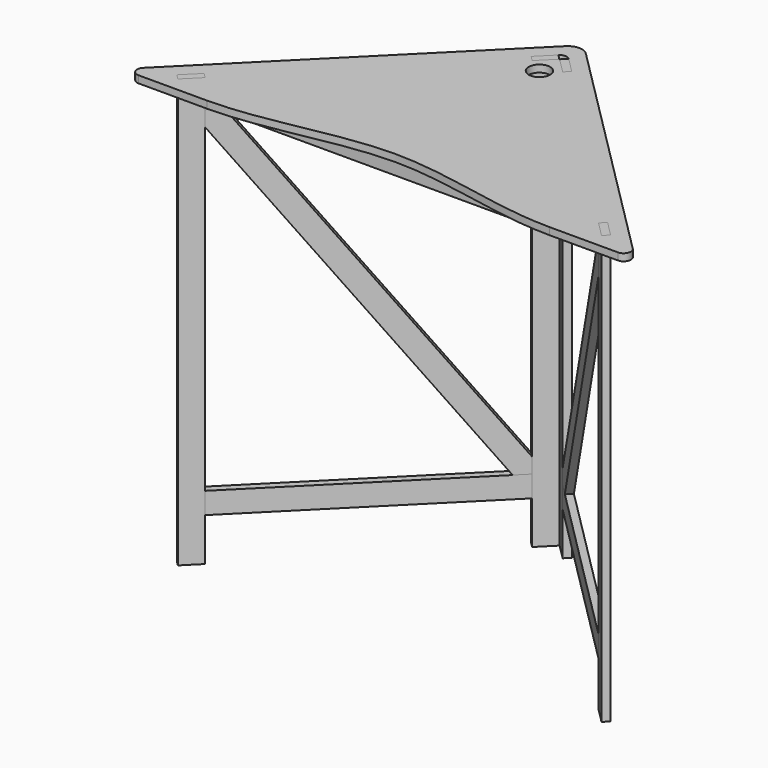
from build123d import *

# Parameters (mm, degrees)
F3_DEPTH  = 12.7
F2_R      = 19.05
F4_DEPTH  = 12.7
F5_DEPTH  = 762
F6_W      = 12.7
F6_H      = 38.1
F7_DEPTH  = 457.1994660567
F9_DEPTH  = 12.7
F11_W     = 12.7
F11_H     = 38.1
F12_REACH = 479.401414142
F13_REACH = 479.401414142


with BuildPart() as f3:
    # F1 (on Top) → F3 (new body)
    with BuildSketch(Plane.XY):
        with BuildLine():
            Line((435.5197438789, 21.6802561211), (17.9605122421, 439.2394877579))
            ThreePointArc((17.9605122421, 439.2394877579), (0, 446.6789755157), (-17.9605122421, 439.2394877579))
            Line((-17.9605122421, 439.2394877579), (-435.5197438789, 21.6802561211))
            ThreePointArc((-435.5197438789, 21.6802561211), (-438.2727578208, 7.839920409), (-426.5394877579, 0))
            Line((-426.5394877579, 0), (-304.8, 0))
            add(Edge.make_bspline(
                [(-304.8, 0), (-203.2, 0), (0, 76.2), (203.2, 0), (304.8, 0)],
                knots=[0, 0, 0, 0, 0.5, 1, 1, 1, 1], degree=3))
            Line((304.8, 0), (426.5394877579, 0))
            ThreePointArc((426.5394877579, 0), (438.2727578208, 7.839920409), (435.5197438789, 21.6802561211))
        make_face()
    extrude(amount=-F3_DEPTH)

    # F2 (on Top) → F4 (cut, through all)
    with BuildSketch(Plane.XY):
        Polygon((-27.1947683632, 376.1236949104), (-0.254, 403.0644632736), (-9.2342561211, 412.0447193947), (-36.1750244843, 385.1039510314), align=None)
        with BuildLine():
            Line((-9.2342561211, 412.0447193947), (-0.254, 403.0644632736))
            ThreePointArc((-0.254, 403.0644632736), (0, 403.1696735184), (0.254, 403.0644632736))
            Line((0.254, 403.0644632736), (9.2342561211, 412.0447193947))
            ThreePointArc((9.2342561211, 412.0447193947), (0, 415.8696735184), (-9.2342561211, 412.0447193947))
        make_face()
        Polygon((9.2342561211, 412.0447193947), (0.254, 403.0644632736), (27.1947683632, 376.1236949104), (36.1750244843, 385.1039510314), align=None)
        Polygon((-358.9697835442, 61.3210244843), (-385.9105519074, 34.3802561211), (-376.9302957863, 25.4), (-349.9895274231, 52.3407683632), align=None)
        Polygon((358.9697835442, 61.3210244843), (349.9895274231, 52.3407683632), (376.9302957863, 25.4), (385.9105519074, 34.3802561211), align=None)
        with Locations((0, 358.4171826682)):
            Circle(F2_R)
    extrude(amount=-F4_DEPTH, mode=Mode.SUBTRACT)


with BuildPart() as f5:
    # F2 (on Top) → F5 (new body)
    with BuildSketch(Plane.XY):
        Polygon((-358.9697835442, 61.3210244843), (-385.9105519074, 34.3802561211), (-376.9302957863, 25.4), (-349.9895274231, 52.3407683632), align=None)
    extrude(amount=-F5_DEPTH)


with BuildPart() as f5b:
    # F2 (on Top) → F5, piece 2 (new body)
    with BuildSketch(Plane.XY):
        Polygon((358.9697835442, 61.3210244843), (349.9895274231, 52.3407683632), (376.9302957863, 25.4), (385.9105519074, 34.3802561211), align=None)
    extrude(amount=-F5_DEPTH)


with BuildPart() as f5c:
    # F2 (on Top) → F5, piece 3 (new body)
    with BuildSketch(Plane.XY):
        Polygon((9.2342561211, 412.0447193947), (0.254, 403.0644632736), (27.1947683632, 376.1236949104), (36.1750244843, 385.1039510314), align=None)
    extrude(amount=-F5_DEPTH)


with BuildPart() as f5d:
    # F2 (on Top) → F5, piece 4 (new body)
    with BuildSketch(Plane.XY):
        Polygon((-27.1947683632, 376.1236949104), (-0.254, 403.0644632736), (-9.2342561211, 412.0447193947), (-36.1750244843, 385.1039510314), align=None)
    extrude(amount=-F5_DEPTH)


with BuildPart() as f7:
    # F6 (on face) → F7 (new body, through all)
    with BuildSketch(Plane(origin=(174.4644632736, 174.4644632736, 0), x_dir=(0.7071067812, -0.7071067812, 0), z_dir=(-0.7071067812, -0.7071067812, 0))):
        with Locations((-291.5392203585, -31.75)):
            Rectangle(F6_W, F6_H)
    extrude(amount=F7_DEPTH)


with BuildPart() as f7b:
    # F6 (on face) → F7, piece 2 (new body, through all)
    with BuildSketch(Plane(origin=(174.4644632736, 174.4644632736, 0), x_dir=(0.7071067812, -0.7071067812, 0), z_dir=(-0.7071067812, -0.7071067812, 0))):
        with Locations((-291.5392203585, -666.75)):
            Rectangle(F6_W, F6_H)
    extrude(amount=F7_DEPTH)


with BuildPart() as f9:
    # F8 (on face) → F9 (new body)
    with BuildSketch(Plane(origin=(-210.6394877579, 210.6394877579, 0), x_dir=(-0.7071067812, -0.7071067812, 0), z_dir=(-0.7071067812, 0.7071067812, 0))):
        Polygon((210.469455943, -78.0025485289), (210.469455943, -50.8), (183.2669074141, -50.8), (-246.7300101136, -620.4974514711), (-246.7300101136, -647.7), (-219.5274615847, -647.7), align=None)
    extrude(amount=-F9_DEPTH)


with BuildPart() as f10_1:
    # F10: instance of F7b
    add(f7b.part.mirror(Plane.YZ))


with BuildPart() as f10_2:
    # F10: instance of F7
    add(f7.part.mirror(Plane.YZ))


with BuildPart() as f10_3:
    # F10: instance of F9
    add(f9.part.mirror(Plane.YZ))


with BuildPart() as f12:
    f12_end = f7.part.faces().sort_by_distance((-188.839189765, 214.4792735086, -31.75))[0]
    # F11 (on Right) → F12 (new body, up to a face of F7 that its end follows)
    with BuildSketch(Plane.YZ):
        with Locations((69.85, -31.75)):
            Rectangle(F11_W, F11_H)
    f12_long = extrude(amount=-F12_REACH, mode=Mode.PRIVATE)
    add(split(f12_long, bisect_by=f12_end, keep=Keep.TOP, mode=Mode.PRIVATE))

    f13_end = f10_2.part.faces().sort_by_distance((188.839189765, 214.4792735086, -31.75))[0]
    # F11 (on Right) → F13 (join, up to a face of F10_2 that its end follows)
    with BuildSketch(Plane.YZ):
        with Locations((69.85, -31.75)):
            Rectangle(F11_W, F11_H)
    f13_long = extrude(amount=F13_REACH, mode=Mode.PRIVATE)
    add(split(f13_long, bisect_by=f13_end, keep=Keep.TOP, mode=Mode.PRIVATE))


solid = Compound([f3.part, f5.part, f5b.part, f5c.part, f5d.part, f7.part, f7b.part, f9.part, f10_1.part, f10_2.part, f10_3.part, f12.part])
